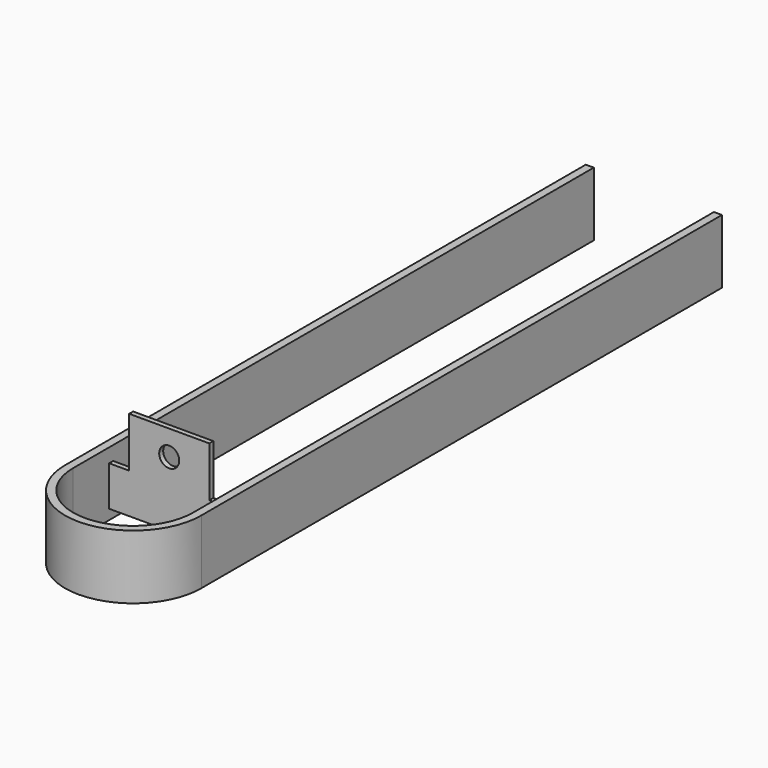
from build123d import *

# Parameters (mm, degrees)
F1_DEPTH  = 1625.6
F3_DEPTH  = 127
F5_D      = 508
F5_DEPTH  = 127
F5_TIP    = 152.618597233
F7_DEPTH  = 15240
F9_DEPTH  = 127
F11_D     = 381
F11_DEPTH = 127
F11_TIP   = 114.4639479248


# Not quite as in the source:
# - a feature names something its author has since deleted; it is built from what else it names


with BuildPart() as f1:
    # F0 (on Top) → F1 (new body)
    with BuildSketch(Plane.XY):
        with BuildLine():
            Line((-1524, 0), (-1727.2, 0))
            Line((-1727.2, 0), (-1727.2, -1270))
            ThreePointArc((-1727.2, -1270), (0, -2997.2), (1727.2, -1270))
            Line((1727.2, -1270), (1727.2, 0))
            Line((1727.2, 0), (1524, 0))
            Line((1524, 0), (1524, -1270))
            ThreePointArc((1524, -1270), (0, -2794), (-1524, -1270))
            Line((-1524, -1270), (-1524, 0))
        make_face()
    extrude(amount=F1_DEPTH)

    # F2 (on Front) → F3 (join)
    with BuildSketch(Plane.XZ):
        Polygon((-1016, 1270), (-1524, 1270), (-1524, 254), (1524, 254), (1524, 1270), (1016, 1270), (1016, 2540), (0, 2540), (-1016, 2540), align=None)
    extrude(amount=F3_DEPTH)

    # F5
    with Locations(Plane(origin=(0, 0, 0), x_dir=(-1, 0, 0), z_dir=(0, 1, 0))):
        with Locations((0, 1905)):
            Hole(F5_D / 2, depth=F5_DEPTH)
            with Locations((0, 0, -(F5_DEPTH + F5_TIP / 2))):  # 118° drill point
                Cone(0, F5_D / 2, F5_TIP, mode=Mode.SUBTRACT)

    # F6 (on face) → F7 (join)
    with BuildSketch(Plane(origin=(0, 0, 0), x_dir=(-1, 0, 0), z_dir=(0, 1, 0))):
        Polygon((-1524, 1270), (-1524, 1625.6), (-1727.2, 1625.6), (-1727.2, 0), (-1524, 0), (-1524, 254), align=None)
        Polygon((1524, 1270), (1524, 254), (1524, 0), (1727.2, 0), (1727.2, 1625.6), (1524, 1625.6), align=None)
    extrude(amount=F7_DEPTH)

    # F8 (on face) → F9 (join)
    with BuildSketch(Plane(origin=(0, 0, 0), x_dir=(1, 0, 0), z_dir=(0, 0, -1))):
        with BuildLine():
            ThreePointArc((-1243.9406885357, 2150.4473654939), (-1452.2984557811, 1731.9580017012), (-1524, 1270))
            Line((-1524, 1270), (1524, 1270))
            ThreePointArc((1524, 1270), (1452.2984557811, 1731.9580017012), (1243.9406885357, 2150.4473654939))
            Line((1243.9406885357, 2150.4473654939), (-1243.9406885357, 2150.4473654939))
        make_face()
    extrude(amount=-F9_DEPTH)

    # F11
    with Locations(Plane.XY.offset(127)):
        with Locations((0, -1701.8)):
            Hole(F11_D / 2, depth=F11_DEPTH)
            with Locations((0, 0, -(F11_DEPTH + F11_TIP / 2))):  # 118° drill point
                Cone(0, F11_D / 2, F11_TIP, mode=Mode.SUBTRACT)


solid = f1.part
